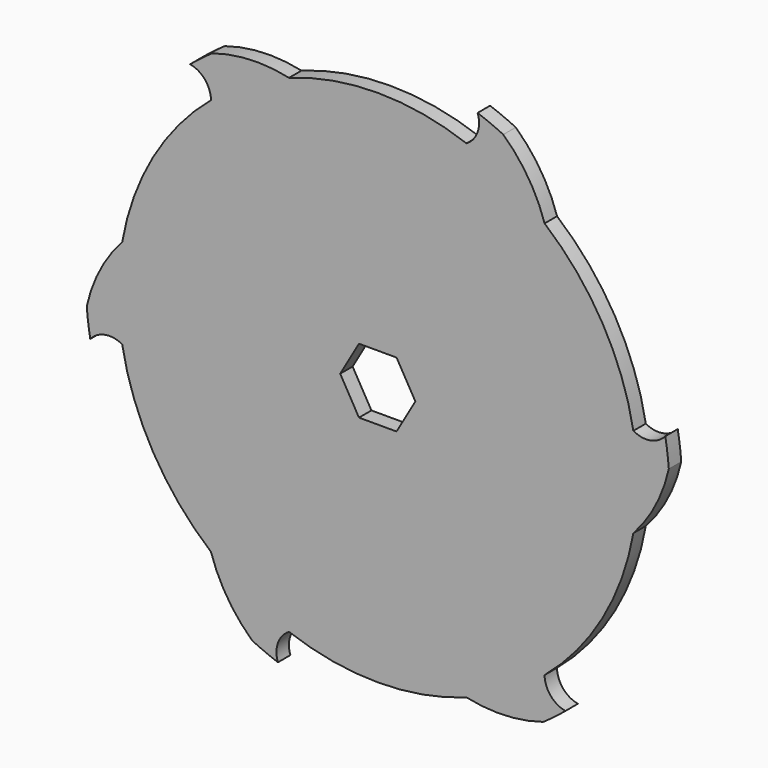
from build123d import *

# Parameters (mm, degrees)
F0_R            = 50.00625
F1_DEPTH        = 1.3335
F3_DEPTH        = 25.4
F3_DEPTH_BACK   = 25.4
F3_COPIES_COUNT = 6


# Not quite as in the source:
# - a pattern or mirror of a feature is missing from the dataset's text; its kind, count and spacing are read off the source's solid


with BuildPart() as f1:
    # F0 (on Front) → F1 (new body, symmetric)
    with BuildSketch(Plane.XZ):
        Circle(F0_R)
        Polygon((-6.4378019116, 0), (-3.2189009558, 5.5753), (3.2189009558, 5.5753), (6.4378019116, 0), (3.2189009558, -5.5753), (-3.2189009558, -5.5753), align=None, mode=Mode.SUBTRACT)
    extrude(amount=F1_DEPTH, both=True)

    # F2 (on Front) → F3 (cut, two sides)
    with BuildSketch(Plane.XZ) as f3_sk:
        with BuildLine():
            ThreePointArc((-15.2027953708, 41.7693369939), (0, 44.45), (15.2027953708, 41.7693369939))
            ThreePointArc((15.2027953708, 41.7693369939), (17.088416716, 44.0394458254), (17.1031447922, 46.9905041182))
            ThreePointArc((17.1031447922, 46.9905041182), (-6.3285699036, 49.6041756512), (-28.3534749263, 41.1910851844))
            ThreePointArc((-28.3534749263, 41.1910851844), (-21.816245393, 42.3469193359), (-15.2027953708, 41.7693369939))
        make_face()
    f3 = extrude(amount=-F3_DEPTH, mode=Mode.SUBTRACT) + extrude(f3_sk.sketch, amount=F3_DEPTH_BACK, mode=Mode.SUBTRACT)

    # F3_copies: F3 ×6 about axis
    f3_copies_axis = Axis((0, 0, 0), (0, 1, 0))
    for i in range(1, F3_COPIES_COUNT):
        add(f3.rotate(f3_copies_axis, i * 360 / F3_COPIES_COUNT), mode=Mode.SUBTRACT)


solid = f1.part
